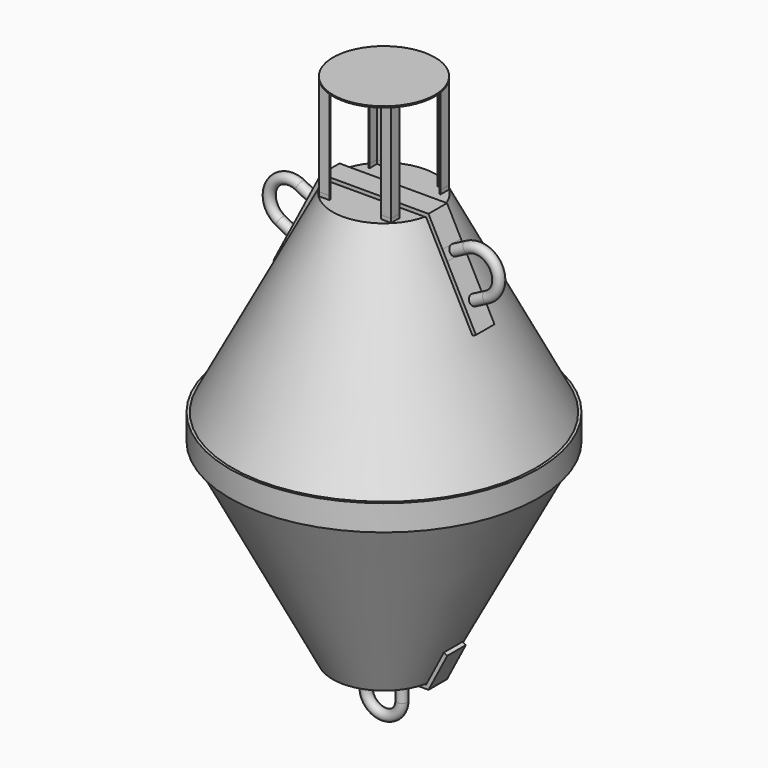
from build123d import *

# Parameters (mm, degrees)
F1_DEPTH  = 45
F2_R      = 20
F3_DEPTH  = 100
F4_R      = 20
F5_ANGLE  = 180
F7_DEPTH  = 60
F8_R      = 19.9999998707
F9_ANGLE  = 180
F10_R     = 19.9999998707
F10_R_2   = 20.0000001013
F11_DEPTH = 60
F12_R     = 19.9999998707
F13_ANGLE = 180
F15_DEPTH = 380
F16_COUNT = 4
F17_R     = 197.9898987322
F18_DEPTH = 5
F20_DEPTH = 15


# Not quite as in the source:
# - ends of sketch curves that miss each other by under 0.0002 mm in the source are joined


with BuildPart() as f1:
    # F0 (on Front) → F1 (new body, symmetric)
    with BuildSketch(Plane.XZ):
        Polygon((-300, 702.5), (-100, 702.5), (80.3396461889, 355.6929880982), (93.647898, 362.61328), (57.893060877, 431.372581936), (39.4389512706, 466.8612541407), (-18.230140877, 577.763354064), (-36.6842502706, 613.2520258593), (-90.893197, 717.5), (-160, 717.5), (-200, 717.5), (-300, 717.5), align=None)
        Polygon((-500, 702.5), (-300, 702.5), (-300, 717.5), (-400, 717.5), (-440, 717.5), (-509.106803, 717.5), (-563.3157497294, 613.2520258593), (-581.769859, 577.763354), (-639.4389512706, 466.8612541407), (-657.893061, 431.372582), (-693.647898, 362.61328), (-680.339646, 355.692988), align=None)
    extrude(amount=F1_DEPTH, both=True)

    # F6 (on face) → F7 (join)
    with BuildSketch(Plane(origin=(-694.4323071411, 0, 361.1048008874), x_dir=(0, -1, 0), z_dir=(-0.8872168006, 0, 0.4613527378))):
        with BuildLine():
            ThreePointArc((19.9999998707, 264.20023709), (-14.1421355323, 278.3423726223), (0, 244.2002372193))
            ThreePointArc((0, 244.2002372193), (14.1421355323, 250.0581015577), (19.9999998707, 264.20023709))
        make_face()
        with BuildLine():
            ThreePointArc((6.11e-08, 119.2002373933), (-14.142135717, 85.0581016181), (20.0000001013, 99.2002372919))
            ThreePointArc((20.0000001013, 99.2002372919), (14.142135717, 113.3423729657), (6.11e-08, 119.2002373933))
        make_face()
    extrude(amount=F7_DEPTH)

    # F8 (on face) → F9 (revolve)
    with BuildSketch(Plane(origin=(-747.6653151783, 0, 388.7859651568), x_dir=(0, -1, 0), z_dir=(-0.8872168006, 0, 0.4613527378))):
        with Locations((0, 264.20023709)):
            Circle(F8_R)
    revolve(axis=Axis((-663.8374132872, 43.6869002879, 549.9934682694), (0, -1, 0)), revolution_arc=F9_ANGLE)

    # F10 (on face) → F11 (join)
    with BuildSketch(Plane(origin=(222.140116359, 0, 115.5128608822), x_dir=(0, 1, 0), z_dir=(0.8872168006, 0, 0.4613527378))):
        with Locations((0, 541.0118797836)):
            Circle(F10_R)
        with Locations((0, 376.0118799856)):
            Circle(F10_R_2)
    extrude(amount=F11_DEPTH)

    # F12 (on face) → F13 (revolve)
    with BuildSketch(Plane(origin=(275.3731243962, 0, 143.1940251516), x_dir=(0, 1, 0), z_dir=(0.8872168006, 0, 0.4613527378))):
        with Locations((0, 541.0118797836)):
            Circle(F12_R)
    revolve(axis=Axis((63.8374132872, -29.2952340096, 549.9934682694), (0, 1, 0)), revolution_arc=F13_ANGLE)


with BuildPart() as f1b:
    # F0 (on Front) → F1, piece 2 (new body, symmetric)
    with BuildSketch(Plane.XZ):
        Polygon((-17.835721, -772.004855), (-31.143973, -765.084564), (-100, -897.5), (-300, -897.5), (-300, -912.5), (-250, -912.5), (-230, -912.5), (-210, -912.5), (-90.893197, -912.5), align=None)
        Polygon((-300, -912.5), (-300, -897.5), (-500, -897.5), (-568.8560267796, -765.0845638854), (-582.164279, -772.004855), (-509.106803, -912.5), (-390, -912.5), (-370, -912.5), (-350, -912.5), align=None)
    extrude(amount=F1_DEPTH, both=True)

    # F2 (on face) → F3 (join)
    with BuildSketch(Plane(origin=(0, 0, -912.5), x_dir=(1, 0, 0), z_dir=(0, 0, -1))):
        with Locations((-230, 0)):
            Circle(F2_R)
        with Locations((-370, 0)):
            Circle(F2_R)
    extrude(amount=F3_DEPTH)

    # F4 (on face) → F5 (revolve)
    with BuildSketch(Plane(origin=(0, 0, -1012.5), x_dir=(1, 0, 0), z_dir=(0, 0, -1))):
        with Locations((-230, 0)):
            Circle(F4_R)
    revolve(axis=Axis((-300, -77.0701915026, -1012.5), (0, 1, 0)), revolution_arc=F5_ANGLE)


with BuildPart() as f15:
    # F14 (on face) → F15 (new body)
    with BuildSketch(Plane.XY.offset(717.5)):
        Polygon((-160, 100), (-160, 140), (-200, 140), (-200, 136), (-164, 136), (-164, 100), align=None)
    extrude(amount=F15_DEPTH)


with BuildPart() as f16_1:
    # F16: instance of F15
    add(f15.part.rotate(Axis((-300, 0, -20.3888225555), (0, 0, -1)), 1 * 360 / F16_COUNT))


with BuildPart() as f16_2:
    # F16: instance of F15
    add(f15.part.rotate(Axis((-300, 0, -20.3888225555), (0, 0, -1)), 2 * 360 / F16_COUNT))


with BuildPart() as f16_3:
    # F16: instance of F15
    add(f15.part.rotate(Axis((-300, 0, -20.3888225555), (0, 0, -1)), 3 * 360 / F16_COUNT))


with BuildPart() as f18:
    # F17 (on face) → F18 (new body)
    with BuildSketch(Plane.XY.offset(1097.5)):
        with Locations((-300, 0)):
            Circle(F17_R)
    extrude(amount=F18_DEPTH)


with BuildPart() as f19:
    # F0 (on Front) → F19 (revolve)
    with BuildSketch(Plane.XZ):
        Polygon((80.3396461889, 355.6929880982), (-100, 702.5), (-300, 702.5), (-300, 697.5), (-103.035601, 697.5), (285, -48.72231), (285, -146.27769), (-9.955601, -713.5), (-300, -713.5), (-300, -721.5), (-14.115601, -721.5), (-103.035601, -892.5), (-300, -892.5), (-300, -897.5), (-100, -897.5), (-31.1439732204, -765.0845638854), (290, -147.5), (300, -147.5), (300, -47.5), (290, -47.5), align=None)
    revolve(axis=Axis((-300, 0, -20.3888225555), (0, 0, -1)))


with BuildPart() as f20:
    # F20 (new, through all): a face of the model
    f20_faces = [f15.part.faces().sort_by_distance(p)[0] for p in [
        (-160.5656854249, 120, 717.5),
    ]]
    extrude(f20_faces, amount=F20_DEPTH)


with BuildPart() as f20b:
    # F20#2 (new, through all): a face of the model
    f20_2_faces = [f16_3.part.faces().sort_by_distance(p)[0] for p in [
        (-420, 139.4343145751, 717.5),
    ]]
    extrude(f20_2_faces, amount=F20_DEPTH)


with BuildPart() as f20c:
    # F20#3 (new, through all): a face of the model
    f20_3_faces = [f16_2.part.faces().sort_by_distance(p)[0] for p in [
        (-439.4343145751, -120, 717.5),
    ]]
    extrude(f20_3_faces, amount=F20_DEPTH)


with BuildPart() as f20d:
    # F20#4 (new, through all): a face of the model
    f20_4_faces = [f16_1.part.faces().sort_by_distance(p)[0] for p in [
        (-180, -139.4343145751, 717.5),
    ]]
    extrude(f20_4_faces, amount=F20_DEPTH)


solid = Compound([f1.part, f1b.part, f15.part, f16_1.part, f16_2.part, f16_3.part, f18.part, f19.part, f20.part, f20b.part, f20c.part, f20d.part])
